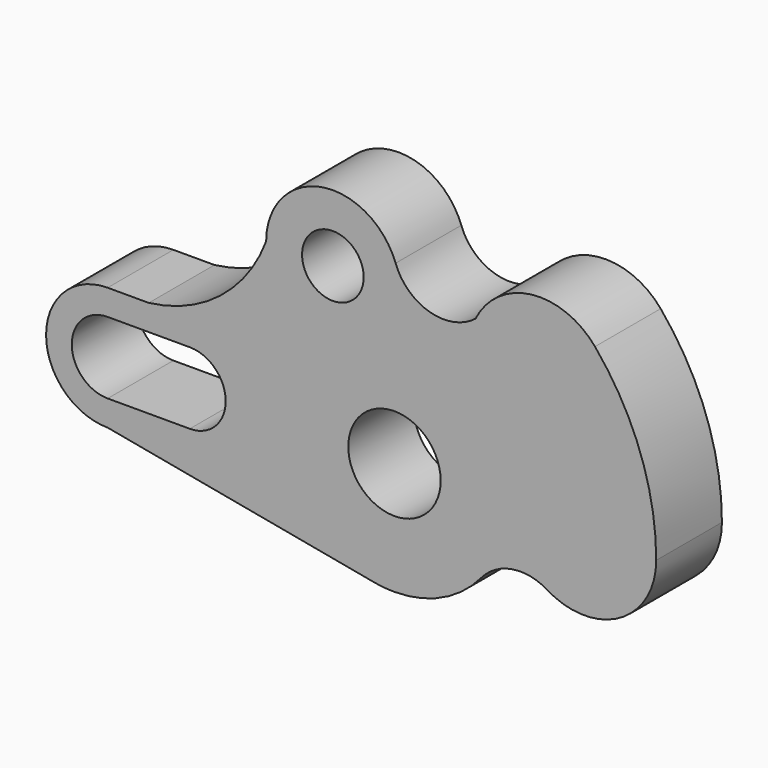
from build123d import *

# Parameters (mm, degrees)
F0_R     = 22.225
F0_R_2   = 14.2875
F0_R_3   = 9.525
F1_DEPTH = 12.7


# Not quite as in the source:
# - the program builds the solid bodies; features that only make, move or delete a surface that nothing else refers to are left out


with BuildPart() as f1:
    # F0 (on Front) → F1 (new body, symmetric)
    with BuildSketch(Plane.XZ):
        with BuildLine():
            ThreePointArc((0.3447838863, 54.6782803896), (1.274446594, 51.2059603319), (1.5875, 47.625))
            ThreePointArc((1.5875, 47.625), (-19.05, 26.9875), (-39.6875, 47.625))
            ThreePointArc((-39.6875, 47.625), (-53.8375681408, 28.2490113175), (-75.9968, 19.05))
            Line((-75.9968, 19.05), (-63.2968, 19.05))
            ThreePointArc((-63.2968, 19.05), (-44.2468, 0), (-63.2968, -19.05))
            Line((-63.2968, -19.05), (-88.6968, -19.05))
            Line((-88.6968, -19.05), (-6.3772739602, -34.3378468245))
            ThreePointArc((-6.3772739602, -34.3378468245), (-3.2021232024, -34.7779019434), (0, -34.925))
            ThreePointArc((0, -34.925), (14.789161423, -31.6391581652), (26.7955113754, -22.3999150697))
            ThreePointArc((26.7955113754, -22.3999150697), (26.830059594, -22.3587292729), (26.8647470812, -22.3176607024))
            ThreePointArc((26.8647470812, -22.3176607024), (36.4241213525, -16.9130263167), (47.2042520761, -19.005988544))
            ThreePointArc((47.2042520761, -19.005988544), (69.6313679155, -19.3648496329), (80.9498, 0))
            ThreePointArc((80.9498, 0), (76.0683727679, 27.6867119276), (62.0118668229, 52.0341345797))
            ThreePointArc((62.0118668229, 52.0341345797), (42.3521205548, 59.8164947236), (25.0767563288, 47.625))
            ThreePointArc((25.0767563288, 47.625), (10.9100684584, 44.8375705557), (0.3447838863, 54.6782803896))
        make_face()
        Circle(F0_R, mode=Mode.SUBTRACT)
        with BuildLine():
            Line((-63.2968, 19.05), (-75.9968, 19.05))
            Line((-75.9968, 19.05), (-88.6968, 19.05))
            ThreePointArc((-88.6968, 19.05), (-107.7468, 0), (-88.6968, -19.05))
            Line((-88.6968, -19.05), (-63.2968, -19.05))
            ThreePointArc((-63.2968, -19.05), (-44.2468, 0), (-63.2968, 19.05))
        make_face()
        with BuildLine():
            ThreePointArc((-88.6968, -11.0998), (-99.7966, 0), (-88.6968, 11.0998))
            Line((-88.6968, 11.0998), (-63.2968, 11.0998))
            ThreePointArc((-63.2968, 11.0998), (-52.197, 0), (-63.2968, -11.0998))
            Line((-63.2968, -11.0998), (-88.6968, -11.0998))
        make_face(mode=Mode.SUBTRACT)
        Circle(F0_R)
        Circle(F0_R_2, mode=Mode.SUBTRACT)
        with BuildLine():
            ThreePointArc((-39.6875, 47.625), (-19.05, 26.9875), (1.5875, 47.625))
            ThreePointArc((1.5875, 47.625), (1.274446594, 51.2059603319), (0.3447838863, 54.6782803896))
            ThreePointArc((0.3447838863, 54.6782803896), (-22.6309603319, 67.949446594), (-39.6875, 47.625))
        make_face()
        with Locations((-19.05, 47.625)):
            Circle(F0_R_3, mode=Mode.SUBTRACT)
    extrude(amount=F1_DEPTH, both=True)


solid = f1.part
